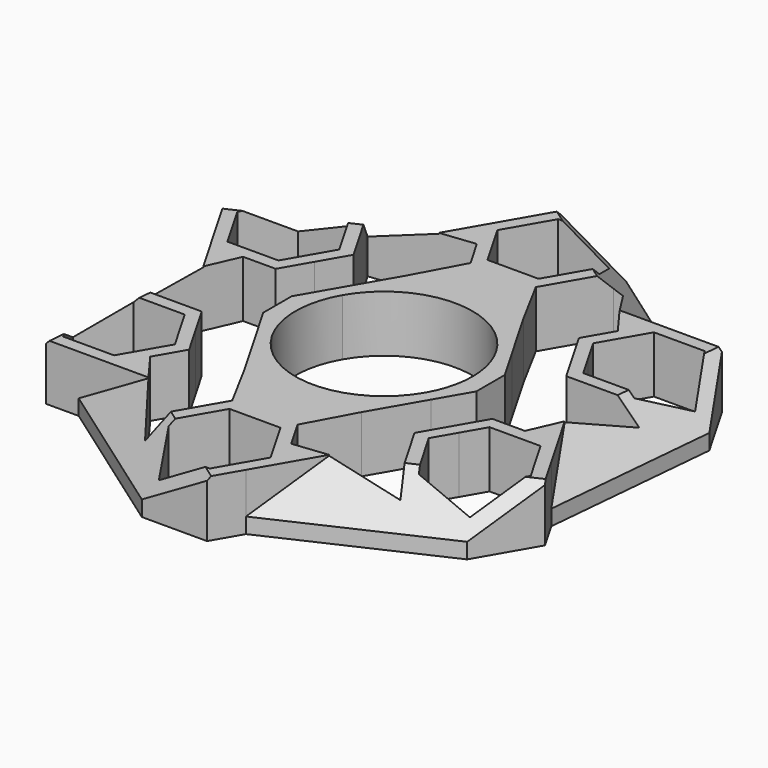
from build123d import *

# Parameters (mm, degrees)
F1_DEPTH     = 6.9977
F2_T4_DEPTH  = 48.1283993469
F2_T9_DEPTH  = 48.1283993469
F2_T14_DEPTH = 48.1283993469
F2_T19_DEPTH = 48.1283993469
F2_T24_DEPTH = 48.1283993469
F2_T29_DEPTH = 48.1283993469
F3_SIZE      = 2.54


# Not quite as in the source:
# - a fillet or chamfer that OpenCascade refuses, or shapes differently, is made with other operations: its cross-section is extruded or revolved along the edge and cut away or added
# - a feature names something its author has since deleted; it is built from what else it names


with BuildPart() as f1:
    # F0 (on Top) → F1 (new body)
    with BuildSketch(Plane.XY):
        Polygon((-13.9314619955, -12.7), (-15.9478578107, -9.2075), (-17.9642536258, -5.715), (-26.0298368864, -5.715), (-30.0626285167, -12.7), (-26.0298368864, -19.685), (-21.9970452561, -19.685), (-17.9642536258, -19.685), (-15.9478578107, -16.1925), align=None)
        Polygon((-18.8441354361, -7.239), (-17.2676805261, -9.9695), (-15.691225616, -12.7), (-18.8441354361, -18.161), (-25.1499550762, -18.161), (-28.3028648962, -12.7), (-25.1499550762, -7.239), align=None, mode=Mode.SUBTRACT)
        with BuildLine():
            ThreePointArc((-9.4807265054, -5.4737), (-10.9474, 0), (-9.4807265054, 5.4737))
            Line((-9.4807265054, 5.4737), (-10.8318467228, 6.2537696213))
            Line((-10.8318467228, 6.2537696213), (-14.4424622971, 0))
            Line((-14.4424622971, 0), (-10.8318467228, -6.2537696213))
            Line((-10.8318467228, -6.2537696213), (-9.4807265054, -5.4737))
        make_face()
        Polygon((-17.9642536258, 5.715), (-15.9478578107, 9.2075), (-13.9314619955, 12.7), (-17.9642536258, 19.685), (-26.0298368864, 19.685), (-30.0626285167, 12.7), (-28.0462327016, 9.2075), (-26.0298368864, 5.715), (-21.9970452561, 5.715), align=None)
        Polygon((-15.691225616, 12.7), (-17.2676805261, 9.9695), (-18.8441354361, 7.239), (-25.1499550762, 7.239), (-28.3028648962, 12.7), (-25.1499550762, 18.161), (-18.8441354361, 18.161), align=None, mode=Mode.SUBTRACT)
        Polygon((-27.0032693489, -5.715), (-21.9970452561, 5.715), (-26.0298368864, 5.715), (-28.0462327016, 9.2075), (-30.0626285167, -12.7), align=None)
        Polygon((-18.4509698571, 20.5280172414), (-6.0491874454, 21.9075), (-8.0655832606, 25.4), (-6.0491874454, 28.8925), (-26.0298368864, 19.685), align=None)
        Polygon((-4.0327916303, 18.415), (4.0327916303, 18.415), (8.0655832606, 25.4), (4.0327916303, 32.385), (-4.0327916303, 32.385), (-6.0491874454, 28.8925), (-8.0655832606, 25.4), (-6.0491874454, 21.9075), align=None)
        Polygon((-6.3058196401, 25.4), (-3.15290982, 30.861), (3.15290982, 30.861), (6.3058196401, 25.4), (3.15290982, 19.939), (-3.15290982, 19.939), align=None, mode=Mode.SUBTRACT)
        Polygon((8.5522994918, 26.2430172414), (15.9478578107, 16.1925), (17.9642536258, 19.685), (21.9970452561, 19.685), (4.0327916303, 32.385), align=None)
        Polygon((27.0032693489, 5.715), (21.9970452561, -5.715), (26.0298368864, -5.715), (28.0462327016, -9.2075), (30.0626285167, 12.7), align=None)
        Polygon((13.9314619955, 12.7), (15.9478578107, 9.2075), (17.9642536258, 5.715), (26.0298368864, 5.715), (30.0626285167, 12.7), (26.0298368864, 19.685), (21.9970452561, 19.685), (17.9642536258, 19.685), (15.9478578107, 16.1925), align=None)
        Polygon((18.8441354361, 7.239), (17.2676805261, 9.9695), (15.691225616, 12.7), (18.8441354361, 18.161), (25.1499550762, 18.161), (28.3028648962, 12.7), (25.1499550762, 7.239), align=None, mode=Mode.SUBTRACT)
        Polygon((18.4509698571, -20.5280172414), (6.0491874454, -21.9075), (8.0655832606, -25.4), (6.0491874454, -28.8925), (26.0298368864, -19.685), align=None)
        Polygon((6.0491874454, -21.9075), (4.0327916303, -18.415), (-4.0327916303, -18.415), (-8.0655832606, -25.4), (-4.0327916303, -32.385), (4.0327916303, -32.385), (6.0491874454, -28.8925), (8.0655832606, -25.4), align=None)
        Polygon((-6.3058196401, -25.4), (-3.15290982, -19.939), (3.15290982, -19.939), (6.3058196401, -25.4), (3.15290982, -30.861), (-3.15290982, -30.861), align=None, mode=Mode.SUBTRACT)
        Polygon((-8.5522994918, -26.2430172414), (-15.9478578107, -16.1925), (-17.9642536258, -19.685), (-21.9970452561, -19.685), (-4.0327916303, -32.385), align=None)
        with BuildLine():
            Line((10.8318467228, -6.2537696213), (9.4807265054, -5.4737))
            ThreePointArc((9.4807265054, -5.4737), (0, -10.9474), (-9.4807265054, -5.4737))
            Line((-9.4807265054, -5.4737), (-10.8318467228, -6.2537696213))
            Line((-10.8318467228, -6.2537696213), (-7.2212311486, -12.5075392425))
            Line((-7.2212311486, -12.5075392425), (7.2212311486, -12.5075392425))
            Line((7.2212311486, -12.5075392425), (10.8318467228, -6.2537696213))
        make_face()
        with BuildLine():
            ThreePointArc((9.4807265054, 5.4737), (10.5743763907, 2.8333956144), (10.9474, 0))
            ThreePointArc((10.9474, 0), (10.5743763907, -2.8333956144), (9.4807265054, -5.4737))
            Line((9.4807265054, -5.4737), (10.8318467228, -6.2537696213))
            Line((10.8318467228, -6.2537696213), (14.4424622971, 0))
            Line((14.4424622971, 0), (10.8318467228, 6.2537696213))
            Line((10.8318467228, 6.2537696213), (9.4807265054, 5.4737))
        make_face()
        with BuildLine():
            ThreePointArc((-9.4807265054, 5.4737), (0, 10.9474), (9.4807265054, 5.4737))
            Line((9.4807265054, 5.4737), (10.8318467228, 6.2537696213))
            Line((10.8318467228, 6.2537696213), (7.2212311486, 12.5075392425))
            Line((7.2212311486, 12.5075392425), (-7.2212311486, 12.5075392425))
            Line((-7.2212311486, 12.5075392425), (-10.8318467228, 6.2537696213))
            Line((-10.8318467228, 6.2537696213), (-9.4807265054, 5.4737))
        make_face()
        Polygon((17.9642536258, -5.715), (15.9478578107, -9.2075), (13.9314619955, -12.7), (17.9642536258, -19.685), (26.0298368864, -19.685), (30.0626285167, -12.7), (28.0462327016, -9.2075), (26.0298368864, -5.715), (21.9970452561, -5.715), align=None)
        Polygon((15.691225616, -12.7), (17.2676805261, -9.9695), (18.8441354361, -7.239), (25.1499550762, -7.239), (28.3028648962, -12.7), (25.1499550762, -18.161), (18.8441354361, -18.161), align=None, mode=Mode.SUBTRACT)
        Polygon((-26.0298368864, 19.685), (-17.9642536258, 19.685), (-18.4509698571, 20.5280172414), align=None)
        Polygon((30.0626285167, 12.7), (26.0298368864, 5.715), (27.0032693489, 5.715), align=None)
        Polygon((26.0298368864, -19.685), (17.9642536258, -19.685), (18.4509698571, -20.5280172414), align=None)
        Polygon((-30.0626285167, -12.7), (-26.0298368864, -5.715), (-27.0032693489, -5.715), align=None)
        Polygon((-7.2212311486, 12.5075392425), (7.2212311486, 12.5075392425), (4.0327916303, 18.415), (-4.0327916303, 18.415), align=None)
        Polygon((4.0327916303, -18.415), (7.2212311486, -12.5075392425), (-7.2212311486, -12.5075392425), (-4.0327916303, -18.415), align=None)
        Polygon((-4.0327916303, -32.385), (-8.0655832606, -25.4), (-8.5522994918, -26.2430172414), align=None)
        Polygon((4.0327916303, 32.385), (8.0655832606, 25.4), (8.5522994918, 26.2430172414), align=None)
    extrude(amount=F1_DEPTH)

    # F2: chamfer of 5.08 on 6 edges, made by hand


with BuildPart() as f2_tool2:
    # F2_s3 → F2_t4 (new body)
    with BuildSketch(Plane(origin=(-1.8021315116, -19.5795864057, 0), x_dir=(0, 0, 1), z_dir=(0.0916539378, 0.9957909197, 0))):
        Polygon((1.9177, 28.7720874875), (6.9977, 23.6920874875), (6.9977, 28.7720874875), align=None)
    extrude(amount=F2_T4_DEPTH)

    split(bisect_by=Plane(origin=(17.0477100735, 9.8425, 0), x_dir=(0, 0, 1), z_dir=(0.8660254038, 0.5, 0)), keep=Keep.TOP)


with BuildPart() as f1_1:
    add(f1.part)

    # F2_t1: cut F2_tool2
    add(f2_tool2.part, mode=Mode.SUBTRACT)


with BuildPart() as f2_tool7:
    # F2_s8 → F2_t9 (new body)
    with BuildSketch(Plane(origin=(16.0553534671, -11.3504848729, 0), x_dir=(0, 0, 1), z_dir=(-0.8165532644, 0.5772700984, 0))):
        Polygon((1.9177, 28.7720874875), (6.9977, 23.6920874875), (6.9977, 28.7720874875), align=None)
    extrude(amount=F2_T9_DEPTH)

    split(bisect_by=Plane.XZ.offset(-19.685), keep=Keep.BOTTOM)


with BuildPart() as f1_2:
    add(f1_1.part)

    # F2_t6: cut F2_tool7
    add(f2_tool7.part, mode=Mode.SUBTRACT)


with BuildPart() as f2_tool12:
    # F2_s13 → F2_t14 (new body)
    with BuildSketch(Plane(origin=(17.8574849787, 8.2291015328, 0), x_dir=(0, 0, 1), z_dir=(-0.9082072022, -0.4185208213, 0))):
        Polygon((1.9177, 28.7720874875), (6.9977, 23.6920874875), (6.9977, 28.7720874875), align=None)
    extrude(amount=F2_T14_DEPTH)

    split(bisect_by=Plane(origin=(-17.0477100735, 9.8425, 0), x_dir=(0, 0, 1), z_dir=(-0.8660254038, 0.5, 0)), keep=Keep.TOP)


with BuildPart() as f1_3:
    add(f1_2.part)

    # F2_t11: cut F2_tool12
    add(f2_tool12.part, mode=Mode.SUBTRACT)


with BuildPart() as f2_tool17:
    # F2_s18 → F2_t19 (new body)
    with BuildSketch(Plane(origin=(1.8021315116, 19.5795864057, 0), x_dir=(0, 0, 1), z_dir=(-0.0916539378, -0.9957909197, 0))):
        Polygon((1.9177, 28.7720874875), (6.9977, 23.6920874875), (6.9977, 28.7720874875), align=None)
    extrude(amount=F2_T19_DEPTH)

    split(bisect_by=Plane(origin=(-17.0477100735, -9.8425, 0), x_dir=(0, 0, 1), z_dir=(-0.8660254038, -0.5, 0)), keep=Keep.TOP)


with BuildPart() as f1_4:
    add(f1_3.part)

    # F2_t16: cut F2_tool17
    add(f2_tool17.part, mode=Mode.SUBTRACT)


with BuildPart() as f2_tool22:
    # F2_s23 → F2_t24 (new body)
    with BuildSketch(Plane(origin=(-16.0553534671, 11.3504848729, 0), x_dir=(0, 0, 1), z_dir=(0.8165532644, -0.5772700984, 0))):
        Polygon((1.9177, 28.7720874875), (6.9977, 23.6920874875), (6.9977, 28.7720874875), align=None)
    extrude(amount=F2_T24_DEPTH)

    split(bisect_by=Plane.XZ.offset(19.685), keep=Keep.TOP)


with BuildPart() as f1_5:
    add(f1_4.part)

    # F2_t21: cut F2_tool22
    add(f2_tool22.part, mode=Mode.SUBTRACT)


with BuildPart() as f2_tool27:
    # F2_s28 → F2_t29 (new body)
    with BuildSketch(Plane(origin=(-17.8574849787, -8.2291015328, 0), x_dir=(0, 0, 1), z_dir=(0.9082072022, 0.4185208213, 0))):
        Polygon((1.9177, 28.7720874875), (6.9977, 23.6920874875), (6.9977, 28.7720874875), align=None)
    extrude(amount=F2_T29_DEPTH)

    split(bisect_by=Plane(origin=(17.0477100735, -9.8425, 0), x_dir=(0, 0, 1), z_dir=(0.8660254038, -0.5, 0)), keep=Keep.TOP)


with BuildPart() as f1_6:
    add(f1_5.part)

    # F2_t26: cut F2_tool27
    add(f2_tool27.part, mode=Mode.SUBTRACT)

    # F3
    f3_edges = [f1_6.edges().sort_by_distance(p)[0] for p in [
        (-14.442462, 0, 3.49885),
        (14.442462, 0, 3.49885),
    ]]
    chamfer(f3_edges, length=F3_SIZE)


solid = f1_6.part
